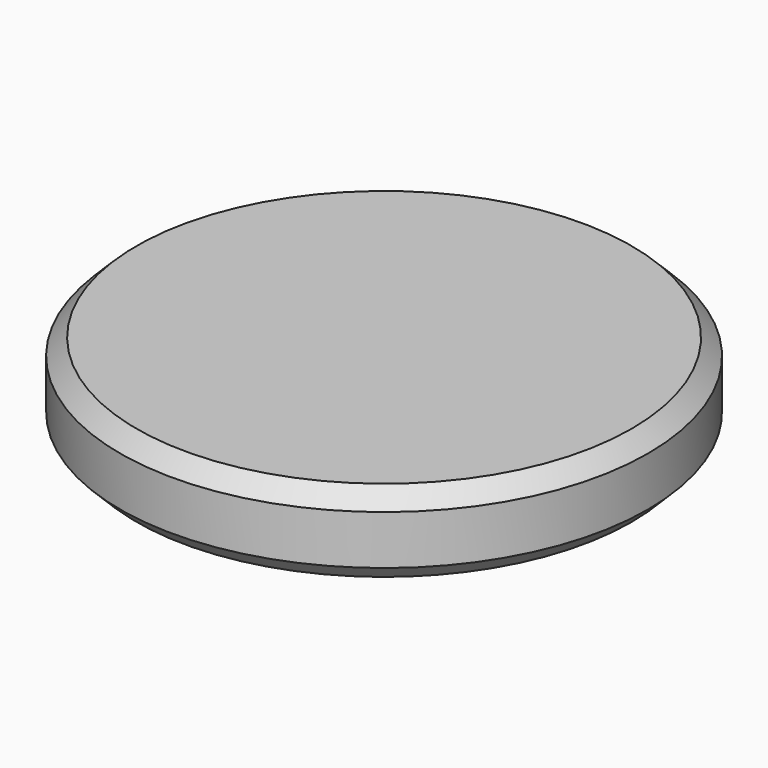
from build123d import *

# Parameters (mm, degrees)
F0_R     = 16.0774395659
F1_DEPTH = 5
F2_SIZE  = 1
F5_SIZE  = 1


# Not quite as in the source:
# - the program builds the solid bodies; features that only make, move or delete a surface that nothing else refers to are left out


with BuildPart() as f1:
    # F0 (on Top) → F1 (new body)
    with BuildSketch(Plane.XY):
        Circle(F0_R)
    extrude(amount=F1_DEPTH)

    # F2
    f2_edges = [f1.edges().sort_by_distance(p)[0] for p in [
        (-16.07744, 0, 5),
    ]]
    chamfer(f2_edges, length=F2_SIZE)

    # F5
    f5_edges = [f1.edges().sort_by_distance(p)[0] for p in [
        (-16.07744, 0, 0),
    ]]
    chamfer(f5_edges, length=F5_SIZE)


solid = f1.part
